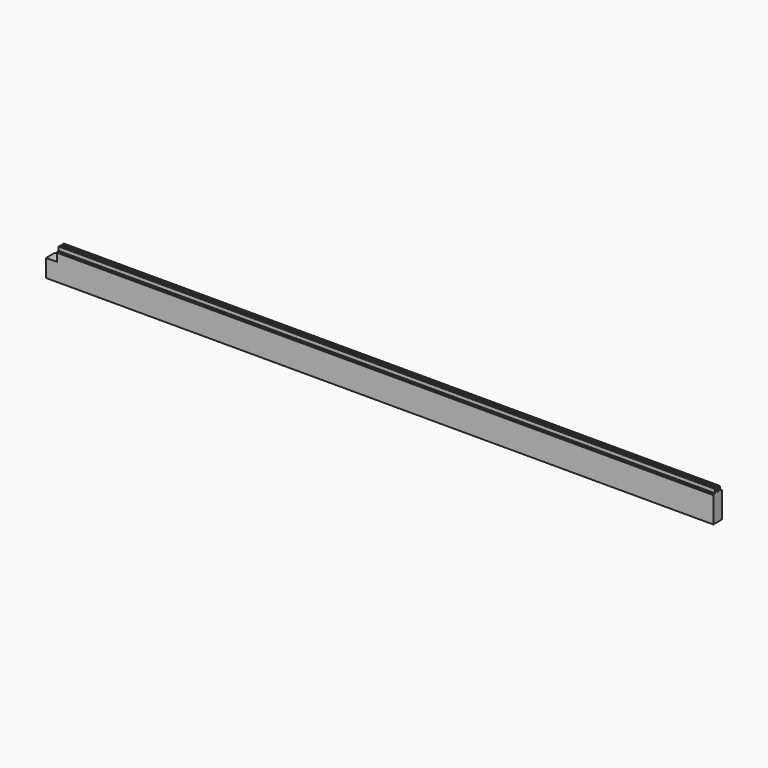
from build123d import *

# Parameters (mm, degrees)
F1_W     = 40
F1_H     = 33
F3_DEPTH = 1240
F2_W     = 80
F2_H     = 100
F4_DEPTH = 25
F5_W     = 2480
F5_H     = 50
F6_DEPTH = 2512


# Not quite as in the source:
# - an extrude ends at something that could not be found from the text; its depth is read off the source's solid


with BuildPart() as f3:
    # F1 (on Right) → F3 (new body, symmetric)
    with BuildSketch(Plane.YZ):
        Polygon((20, 33), (20, 63), (17, 66), (12, 66), (12, 80), (4, 80), (4, 66), (-4, 66), (-4, 80), (-12, 80), (-12, 66), (-17, 66), (-20, 63), (-20, 33), align=None)
        with Locations((0, 16.5)):
            Rectangle(F1_W, F1_H)
        with Locations((0, -16.5)):
            Rectangle(F1_W, F1_H)
    extrude(amount=F3_DEPTH, both=True)

    # F2 (on Front) → F4 (cut, symmetric)
    with BuildSketch(Plane.XZ):
        with Locations((-1240, 83)):
            Rectangle(F2_W, F2_H)
        with Locations((-1240, -83)):
            Rectangle(F2_W, F2_H)
    extrude(amount=F4_DEPTH, both=True, mode=Mode.SUBTRACT)

    # F5 (on face) → F6 (cut, through all)
    with BuildSketch(Plane.XZ.offset(20)):
        with Locations((0, -58)):
            Rectangle(F5_W, F5_H)
    extrude(amount=-F6_DEPTH, mode=Mode.SUBTRACT)


solid = f3.part
